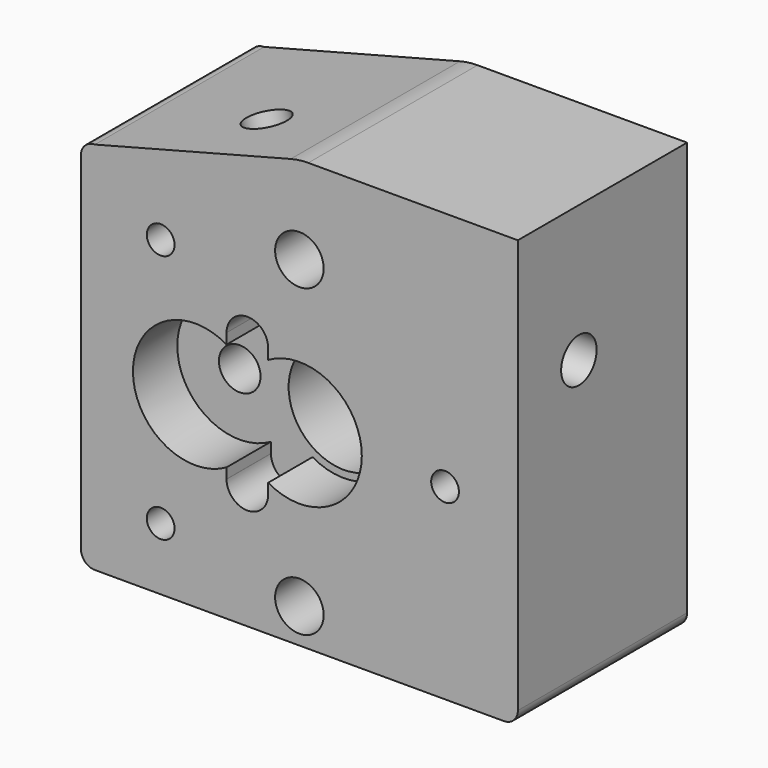
from build123d import *

# Parameters (mm, degrees)
F0_R             = 6
F0_R_2           = 3.975
F1_DEPTH         = 15.25
F2_R             = 6
F2_R_2           = 3.975
F3_DEPTH         = 6.25
F4_R             = 3.975
F5_DEPTH         = 4
F6_R             = 1.5
F7_DEPTH         = 4.5
F8_R             = 1.75
F9_DEPTH         = 15.251
F10_R            = 1
F11_DEPTH        = 15.251
F11_COPIES_COUNT = 2
F11_COPIES_PITCH = 22.388613
F12_R            = 1.7592557298
F12_R_2          = 1
F12_R_3          = 1.75
F13_DEPTH        = 8
F14_R            = 2.1
F15_DEPTH        = 8
F17_DEPTH        = 2
F18_R            = 1.6
F19_DEPTH        = 12
F20_R            = 0.9
F21_DEPTH        = 20
F23_DEPTH        = 15.25
F24_R            = 1.5
F25_DEPTH        = 11


# Not quite as in the source:
# - a pattern or mirror of a feature is missing from the dataset's text; its kind, count and spacing are read off the source's solid
# - a feature names something its author has since deleted; it is built from what else it names


with BuildPart() as f1:
    # F0 (on Front) → F1 (new body)
    with BuildSketch(Plane.XZ):
        with BuildLine():
            Line((-14.75, -13.5), (14.75, -13.5))
            ThreePointArc((14.75, -13.5), (15.4571067812, -13.2071067812), (15.75, -12.5))
            Line((15.75, -12.5), (15.75, 12.5))
            ThreePointArc((15.75, 12.5), (15.4571067812, 13.2071067812), (14.75, 13.5))
            Line((14.75, 13.5), (-14.75, 13.5))
            ThreePointArc((-14.75, 13.5), (-15.4571067812, 13.2071067812), (-15.75, 12.5))
            Line((-15.75, 12.5), (-15.75, -12.5))
            ThreePointArc((-15.75, -12.5), (-15.4571067812, -13.2071067812), (-14.75, -13.5))
        make_face()
        Circle(F0_R, mode=Mode.SUBTRACT)
        Circle(F0_R)
        Circle(F0_R_2, mode=Mode.SUBTRACT)
    extrude(amount=F1_DEPTH)

    # F2 (on face) → F3 (cut)
    with BuildSketch(Plane(origin=(0, 0, 0), x_dir=(-1, 0, 0), z_dir=(0, 1, 0))):
        Circle(F2_R)
        Circle(F2_R_2, mode=Mode.SUBTRACT)
    extrude(amount=-F3_DEPTH, mode=Mode.SUBTRACT)

    # F4 (on face) → F5 (cut)
    with BuildSketch(Plane.XZ.offset(15.25)):
        with BuildLine():
            Line((-2.2497879514, -4.6444608866), (-2.2497871292, -3.8972372103))
            ThreePointArc((-2.2497871292, -3.8972372103), (4.5, -4.9516e-06), (-2.2497785524, 3.8972421615))
            Line((-2.2497785524, 3.8972421615), (-2.2497777241, 4.6499983495))
            ThreePointArc((-2.2497777241, 4.6499983495), (-3.7497777241, 6.15), (-5.2497777241, 4.6499983495))
            Line((-5.2497777241, 4.6499983495), (-5.2497768955, 3.8969854991))
            ThreePointArc((-5.2497768955, 3.8969854991), (-12, -4.9516e-06), (-5.2497683193, -3.8969805469))
            Line((-5.2497683193, -3.8969805469), (-5.2497674968, -4.6444608866))
            ThreePointArc((-5.2497674968, -4.6444608866), (-5.2497777241, -4.6500016505), (-5.2497674846, -4.6555424145))
            ThreePointArc((-5.2497674846, -4.6555424145), (-3.7497777241, -6.15), (-2.2497879636, -4.6555424145))
            ThreePointArc((-2.2497879636, -4.6555424145), (-2.2497777241, -4.6500016505), (-2.2497879514, -4.6444608866))
        make_face()
        Circle(F4_R, mode=Mode.SUBTRACT)
    extrude(amount=-F5_DEPTH, mode=Mode.SUBTRACT)

    # F6 (on face) → F7 (cut)
    with BuildSketch(Plane.XZ.offset(11.25)):
        with Locations((-7.5, 0)):
            Circle(F6_R)
    extrude(amount=-F7_DEPTH, mode=Mode.SUBTRACT)

    # F8 (on face) → F9 (cut, through all)
    with BuildSketch(Plane(origin=(0, 0, 0), x_dir=(-1, 0, 0), z_dir=(0, 1, 0))):
        with Locations((0, -11)):
            Circle(F8_R)
    f9 = extrude(amount=-F9_DEPTH, mode=Mode.SUBTRACT)

    # F9_copies: F9 across plane
    add(f9.mirror(Plane.XY), mode=Mode.SUBTRACT)

    # F10 (on face) → F11 (cut, through all)
    with BuildSketch(Plane(origin=(0, 0, 0), x_dir=(-1, 0, 0), z_dir=(0, 1, 0))):
        with Locations((-10.5, 0)):
            Circle(F10_R)
        with Locations((10, -9)):
            Circle(F10_R)
    f11 = extrude(amount=-F11_DEPTH, mode=Mode.SUBTRACT)

    # F11_copies: F11 ×2
    with Locations(*[Vector(-0.9156440302, 0, 0.401990062) * (i * F11_COPIES_PITCH) for i in range(1, F11_COPIES_COUNT)]):
        add(f11, mode=Mode.SUBTRACT)

    # F12 (on face) → F13 (cut)
    with BuildSketch(Plane(origin=(0, 0, 0), x_dir=(-1, 0, 0), z_dir=(0, 1, 0))):
        with Locations((10, -9)):
            Circle(F12_R)
        with Locations((10, -9)):
            Circle(F12_R_2, mode=Mode.SUBTRACT)
        with Locations((-10.5, 0)):
            Circle(F12_R_3)
        with Locations((-10.5, 0)):
            Circle(F12_R_2, mode=Mode.SUBTRACT)
        with Locations((10, 9)):
            Circle(F12_R_3)
        with Locations((9.9999998377, 8.9999999288)):
            Circle(F12_R_2, mode=Mode.SUBTRACT)
    extrude(amount=-F13_DEPTH, mode=Mode.SUBTRACT)

    # F14 (on face) → F15 (cut)
    with BuildSketch(Plane.XY.offset(13.5)):
        with Locations((5, -9.75)):
            Circle(F14_R)
    extrude(amount=-F15_DEPTH, mode=Mode.SUBTRACT)

    # F16 (on face) → F17 (cut)
    with BuildSketch(Plane.XZ.offset(11.25)):
        with BuildLine():
            ThreePointArc((-5.2497777241, 4.6499983495), (-3.7497768988, 3.15), (-2.2497777241, 4.65))
            ThreePointArc((-2.2497777241, 4.65), (-3.7497785494, 6.15), (-5.2497777241, 4.6499983495))
        make_face()
    extrude(amount=-F17_DEPTH, mode=Mode.SUBTRACT)

    # F18 (on face) → F19 (cut)
    with BuildSketch(Plane.YZ.offset(15.75)):
        with Locations((-9.75, 7.5)):
            Circle(F18_R)
    extrude(amount=-F19_DEPTH, mode=Mode.SUBTRACT)

    # F20 (on face) → F21 (cut)
    with BuildSketch(Plane.YZ.offset(15.75)):
        with Locations((-9.75, 7.5)):
            Circle(F20_R)
    extrude(amount=-F21_DEPTH, mode=Mode.SUBTRACT)

    # F22 (on face) → F23 (join, through all)
    with BuildSketch(Plane.XZ.offset(15.25)):
        with BuildLine():
            Line((-0.6199523885, 17.1813922581), (-14.75, 13.5))
            Line((-14.75, 13.5), (14.75, 13.5))
            ThreePointArc((14.75, 13.5), (15.4571067812, 13.2071067812), (15.75, 12.5))
            Line((15.75, 12.5), (15.75, 17.3429124444))
            Line((15.75, 17.3429124444), (0.6406479022, 17.3429124444))
            ThreePointArc((0.6406479022, 17.3429124444), (0.005194941, 17.3023680128), (-0.6199523885, 17.1813922581))
        make_face()
    extrude(amount=-F23_DEPTH)

    # F24 (on face) → F25 (cut)
    with BuildSketch(Plane(origin=(-4.2312468171, 0, 16.240518475), x_dir=(0.9676959627, 0, 0.2521200581), z_dir=(-0.2521200581, 0, 0.9676959627))):
        with Locations((-2.4117373396, -9.9919419736)):
            Circle(F24_R)
    extrude(amount=-F25_DEPTH, mode=Mode.SUBTRACT)


solid = f1.part
